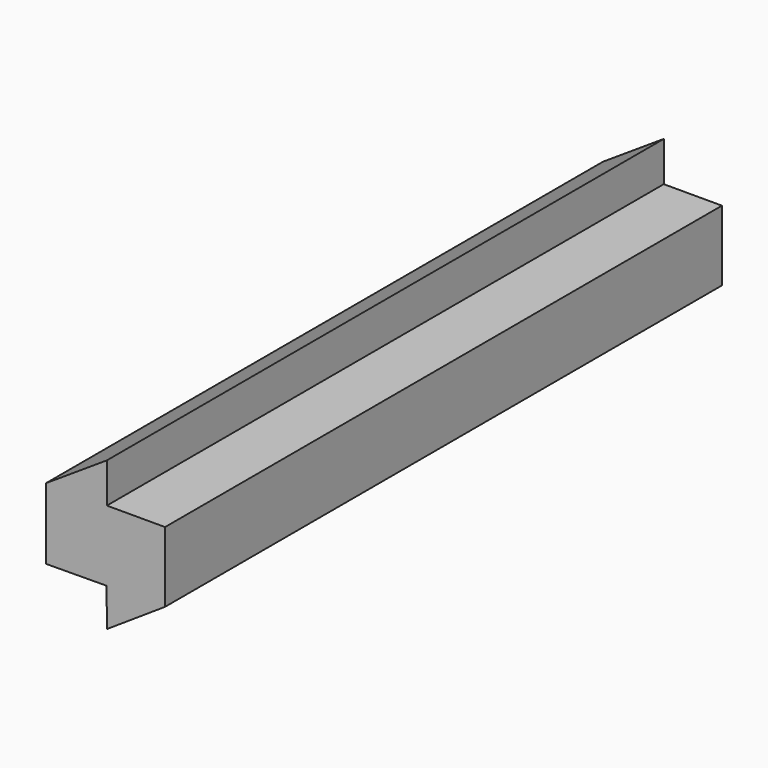
from build123d import *

# Parameters (mm, degrees)
F1_DEPTH = 150


# Not quite as in the source:
# - a feature of the source that left no trace in its solid (it failed there, or was rolled back) is left out


with BuildPart() as f1:
    # F0 (on Front) → F1 (new body)
    with BuildSketch(Plane.XZ):
        Polygon((0.316192396, 10.0656654686), (-12.7883255482, 10.0656654686), (-12.7883255482, -5.258587189), (0.2559647712, -5.1627713866), (12.8449704498, -5.0702998415), (12.8449704498, 10.0656654686), align=None)
        Polygon((0.316192396, 18.6481969431), (-12.7883255482, 10.0656654686), (0.316192396, 10.0656654686), align=None)
        Polygon((12.8449704498, -5.0702998415), (0.2559647712, -5.1627713866), (0.316192396, -13.3621143177), align=None)
    extrude(amount=F1_DEPTH)


solid = f1.part
